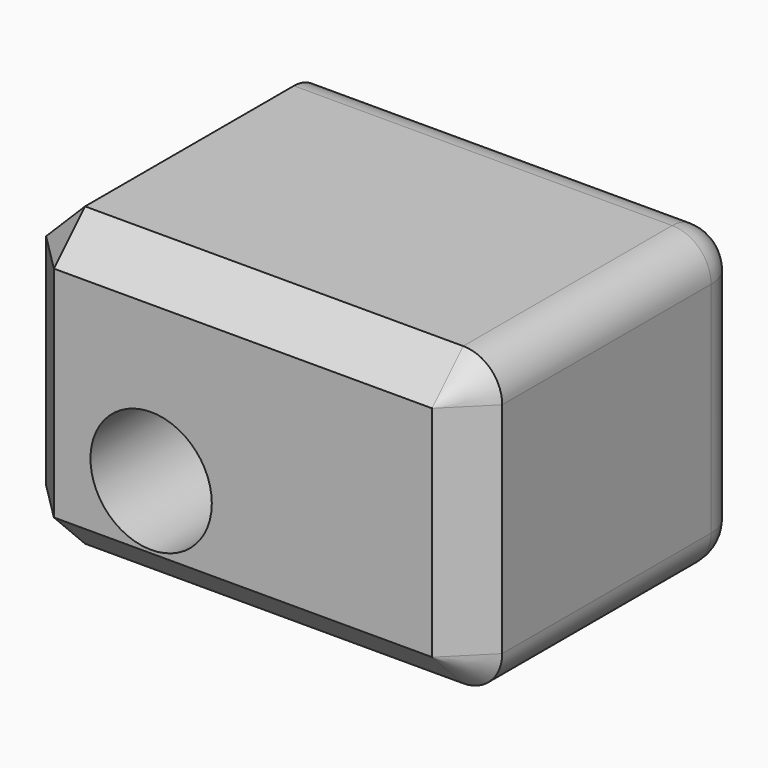
from build123d import *

# Parameters (mm, degrees)
F0_W     = 59.4862774014
F0_H     = 38.7252047658
F1_DEPTH = 44.196
F2_R     = 7.9122216874
F3_DEPTH = 70.104
F4_R     = 5.08
F5_SIZE  = 5.07999


# Not quite as in the source:
# - a fillet or chamfer is up to 0.001 mm smaller than in the source, because OpenCascade refuses the exact size


with BuildPart() as f1:
    # F0 (on Front) → F1 (new body)
    with BuildSketch(Plane.XZ):
        with Locations((29.7431387007, 19.3626023829)):
            Rectangle(F0_W, F0_H)
    extrude(amount=F1_DEPTH)

    # F2 (on face) → F3 (cut)
    with BuildSketch(Plane.XZ.offset(44.196)):
        with Locations((17.7647974342, 13.3899012581)):
            Circle(F2_R)
    extrude(amount=-F3_DEPTH, mode=Mode.SUBTRACT)

    # F4
    f4_edges = [f1.edges().sort_by_distance(p)[0] for p in [
        (59.486277, -22.098, 38.725205),
        (59.486277, -22.098, 0),
        (59.486277, 0, 19.362602),
        (29.743139, 0, 38.725205),
        (29.743139, 0, 0),
    ]]
    fillet(f4_edges, radius=F4_R)

    # F5 (size 5.08 in the source; OpenCascade refuses exactly that, so slightly less here)
    f5_edges = [f1.edges().sort_by_distance(p)[0] for p in [
        (0, -44.196, 19.362602),
        (27.203139, -44.196, 0),
        (0, -24.638, 0),
    ]]
    chamfer(f5_edges, length=F5_SIZE)


solid = f1.part
